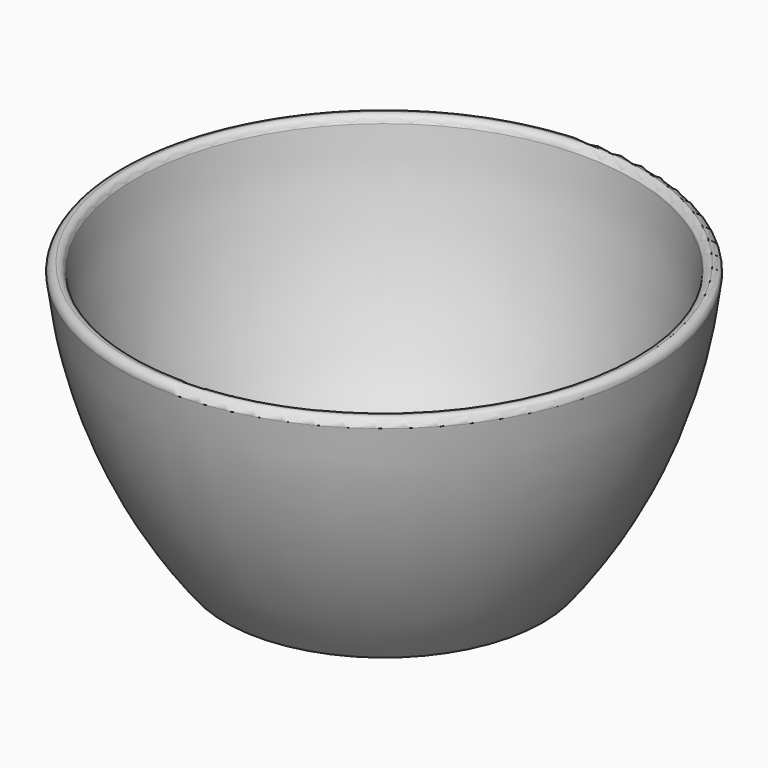
from build123d import *

# Parameters (mm, degrees)
F3_T = -2.88
F4_R = 10


# Not quite as in the source:
# - a fillet or chamfer that OpenCascade refuses, or shapes differently, is made with other operations: its cross-section is extruded or revolved along the edge and cut away or added


with BuildPart() as f2:
    # F1 (on Front) → F2 (revolve)
    with BuildSketch(Plane.XZ):
        with BuildLine():
            Line((0, 50), (0, 0))
            Line((0, 0), (30, 0))
            ThreePointArc((30, 0), (43.6518375699, 23.5392649721), (50, 50))
            Line((50, 50), (0, 50))
        make_face()
    revolve(axis=Axis((0, 0, 25), (0, 0, 1)))

    # F3
    f3_openings = [f2.faces().sort_by_distance(p)[0] for p in [
        (0, 0, 50),
    ]]
    offset(amount=F3_T, openings=f3_openings)

    # F4
    f4_edges = [f2.edges().sort_by_distance(p)[0] for p in [
        (-28.595074, 0, 2.88),
    ]]
    fillet(f4_edges, radius=F4_R)

    # F5: fillet of radius 1.44 on 2 edges, made by hand

    # F5_s1 → F5_t2 (revolve, cut)
    with BuildSketch(Plane.XZ):
        with BuildLine():
            ThreePointArc((48.4100641855, 50), (49.4814986652, 49.5220957102), (49.8417621254, 48.4055946606))
            ThreePointArc((49.8417621254, 48.4055946606), (49.9242734615, 49.2024606493), (50, 50))
            Line((50, 50), (48.4100641855, 50))
        make_face()
    revolve(axis=Axis((0, 0, 50), (0, 0, 1)), mode=Mode.SUBTRACT)

    # F5_s3 → F5_t4 (revolve, cut)
    with BuildSketch(Plane.XZ):
        with BuildLine():
            ThreePointArc((46.9783662426, 48.7144053403), (47.4479684725, 49.63143448), (48.4100641824, 50))
            Line((48.4100641824, 50), (47.1078138243, 50))
            ThreePointArc((47.1078138243, 50), (47.0453655077, 49.3569735508), (46.9783662426, 48.7144053403))
        make_face()
    revolve(axis=Axis((-1.2e-09, -1e-10, 50), (0, 0, -1)), mode=Mode.SUBTRACT)


solid = f2.part
